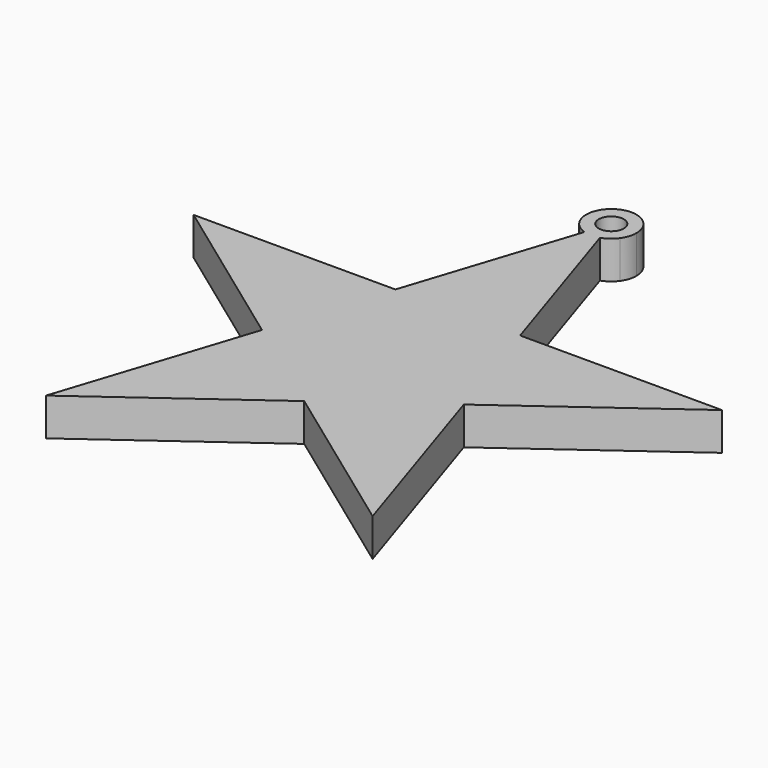
from build123d import *

# Parameters (mm, degrees)
F1_DEPTH = 3


# Not quite as in the source:
# - a feature names something its author has since deleted; it is built from what else it names


with BuildPart() as f1:
    # F0 (on Top) → F1 (new body)
    with BuildSketch(Plane.XY):
        with BuildLine():
            ThreePointArc((0.6180339887, 20.2093431474), (0, 20.11145618), (-0.6180339887, 20.2093431474))
            Line((-0.6180339887, 20.2093431474), (-4.9643312139, 6.83281573))
            Line((-4.9643312139, 6.83281573), (-21.0292444848, 6.83281573))
            Line((-21.0292444848, 6.83281573), (-8.0324566354, -2.60990337))
            Line((-8.0324566354, -2.60990337), (-12.9967878493, -17.88854382))
            Line((-12.9967878493, -17.88854382), (0, -8.44582472))
            Line((0, -8.44582472), (12.9967878493, -17.88854382))
            Line((12.9967878493, -17.88854382), (8.0324566354, -2.60990337))
            Line((8.0324566354, -2.60990337), (21.0292444848, 6.83281573))
            Line((21.0292444848, 6.83281573), (4.9643312139, 6.83281573))
            Line((4.9643312139, 6.83281573), (0.6180339887, 20.2093431474))
        make_face()
        with BuildLine():
            ThreePointArc((0.3090169944, 21.1603996637), (0, 21.11145618), (-0.3090169944, 21.1603996637))
            Line((-0.3090169944, 21.1603996637), (-0.6180339887, 20.2093431474))
            ThreePointArc((-0.6180339887, 20.2093431474), (0, 20.11145618), (0.6180339887, 20.2093431474))
            Line((0.6180339887, 20.2093431474), (0.3090169944, 21.1603996637))
        make_face()
        with BuildLine():
            Line((1.6180339887, 20.9358856754), (0.8090169944, 21.5236709277))
            ThreePointArc((0.8090169944, 21.5236709277), (0.5877852523, 21.3024391856), (0.3090169944, 21.1603996637))
            Line((0.3090169944, 21.1603996637), (0.6180339887, 20.2093431474))
            ThreePointArc((0.6180339887, 20.2093431474), (1.1755705046, 20.4934221913), (1.6180339887, 20.9358856754))
        make_face()
        with BuildLine():
            ThreePointArc((1, 22.11145618), (0.9510565163, 21.8024391856), (0.8090169944, 21.5236709277))
            Line((0.8090169944, 21.5236709277), (1.6180339887, 20.9358856754))
            ThreePointArc((1.6180339887, 20.9358856754), (1.9021130326, 21.4934221913), (2, 22.11145618))
            ThreePointArc((2, 22.11145618), (-0.6180339887, 24.0135692126), (-1.6180339887, 20.9358856754))
            Line((-1.6180339887, 20.9358856754), (-0.8090169944, 21.5236709277))
            ThreePointArc((-0.8090169944, 21.5236709277), (-0.3090169944, 23.0625126963), (1, 22.11145618))
        make_face()
        with BuildLine():
            ThreePointArc((-0.3090169944, 21.1603996637), (-0.5877852523, 21.3024391856), (-0.8090169944, 21.5236709277))
            Line((-0.8090169944, 21.5236709277), (-1.6180339887, 20.9358856754))
            ThreePointArc((-1.6180339887, 20.9358856754), (-1.1755705046, 20.4934221913), (-0.6180339887, 20.2093431474))
            Line((-0.6180339887, 20.2093431474), (-0.3090169944, 21.1603996637))
        make_face()
    extrude(amount=F1_DEPTH)


solid = f1.part
